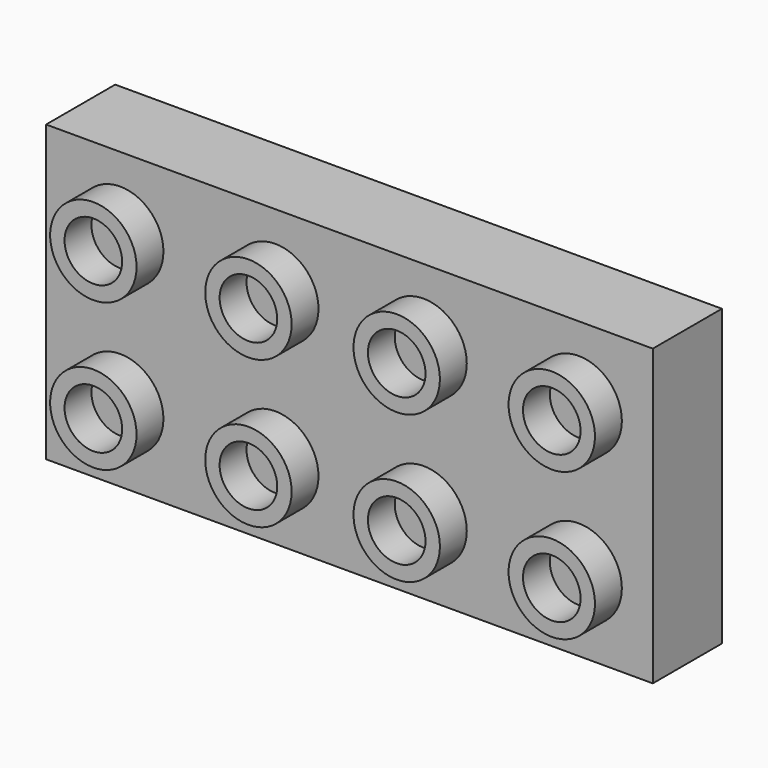
from build123d import *

# Parameters (mm, degrees)
F0_W     = 63.2
F0_H     = 30.7
F1_DEPTH = 9
F2_R     = 4.5
F2_R_2   = 3
F3_DEPTH = 3.5
F4_T     = 1


# Not quite as in the source:
# - a shell that OpenCascade refuses in one call is made with other operations: the cavity is built on its own and cut out


with BuildPart() as f1:
    # F0 (on Front) → F1 (new body)
    with BuildSketch(Plane.XZ):
        with Locations((2.7909118284, 0)):
            Rectangle(F0_W, F0_H)
    extrude(amount=F1_DEPTH)

    # F2 (on face) → F3 (join)
    with BuildSketch(Plane.XZ.offset(9)):
        with Locations((-21.0856401334, 7.675)):
            Circle(F2_R)
        with Locations((-21.0856401334, 7.675)):
            Circle(F2_R_2, mode=Mode.SUBTRACT)
        with Locations((-4.9325362097, 7.675)):
            Circle(F2_R)
        with Locations((-4.9325362097, 7.675)):
            Circle(F2_R_2, mode=Mode.SUBTRACT)
        with Locations((10.5143598666, 7.675)):
            Circle(F2_R)
        with Locations((10.5143598666, 7.675)):
            Circle(F2_R_2, mode=Mode.SUBTRACT)
        with Locations((-4.9325362097, -7.675)):
            Circle(F2_R)
        with Locations((-4.9325362097, -7.675)):
            Circle(F2_R_2, mode=Mode.SUBTRACT)
        with Locations((10.5143598666, -7.675)):
            Circle(F2_R)
        with Locations((10.5143598666, -7.675)):
            Circle(F2_R_2, mode=Mode.SUBTRACT)
        with Locations((-21.0856401334, -7.675)):
            Circle(F2_R)
        with Locations((-21.0856401334, -7.675)):
            Circle(F2_R_2, mode=Mode.SUBTRACT)
        with Locations((26.6674637903, -7.675)):
            Circle(F2_R)
        with Locations((26.6674637903, -7.675)):
            Circle(F2_R_2, mode=Mode.SUBTRACT)
        with Locations((26.6674637903, 7.675)):
            Circle(F2_R)
        with Locations((26.6674637903, 7.675)):
            Circle(F2_R_2, mode=Mode.SUBTRACT)
    extrude(amount=F3_DEPTH)

    # F4: shell of thickness 1, made by hand


with BuildPart() as f4_core1:
    # F4_t2: copy of F1
    add(f1.part)

    # the walls: a layer under each face that stays
    f4_faces = [f4_core1.faces().sort_by_distance(p)[0] for p in [
        (2.7909118284, -4.5, -15.35),
        (-28.8090881716, -4.5, 0),
        (34.3909118284, -4.5, 0),
        (2.7909118284, -9, 0),
        (2.7909118284, -4.5, 15.35),
        (-25.5856401334, -10.75, -7.675),
        (-9.4325362097, -10.75, -7.675),
        (6.0143598666, -10.75, -7.675),
        (22.1674637903, -10.75, -7.675),
        (-25.5856401334, -10.75, 7.675),
        (-9.4325362097, -10.75, 7.675),
        (6.0143598666, -10.75, 7.675),
        (22.1674637903, -10.75, 7.675),
        (-24.0856401334, -12.5, -10.675),
        (-7.9325362097, -12.5, -10.675),
        (7.5143598666, -12.5, -10.675),
        (23.6674637903, -12.5, -10.675),
        (-24.0856401334, -12.5, 4.675),
        (-7.9325362097, -12.5, 4.675),
        (7.5143598666, -12.5, 4.675),
        (23.6674637903, -12.5, 4.675),
        (-24.0856401334, -10.75, -7.675),
        (-7.9325362097, -10.75, -7.675),
        (7.5143598666, -10.75, -7.675),
        (23.6674637903, -10.75, -7.675),
        (-24.0856401334, -10.75, 7.675),
        (-7.9325362097, -10.75, 7.675),
        (7.5143598666, -10.75, 7.675),
        (23.6674637903, -10.75, 7.675),
        (-21.0856401334, -9, -7.675),
        (-4.9325362097, -9, -7.675),
        (10.5143598666, -9, -7.675),
        (26.6674637903, -9, -7.675),
        (-21.0856401334, -9, 7.675),
        (-4.9325362097, -9, 7.675),
        (10.5143598666, -9, 7.675),
        (26.6674637903, -9, 7.675),
    ]]
    thicken(f4_faces, amount=-F4_T, mode=Mode.SUBTRACT)

    # F4_s3 → F4_t4 (revolve, cut)
    with BuildSketch(Plane.XY.offset(-7.675)):
        Polygon((-16.5756401334, -9.01), (-16.5856401334, -8), (-17.5856401334, -8), (-17.5856401334, -9), align=None)
    revolve(axis=Axis((-21.0856401334, -9, -7.675), (0, -1, 0)), mode=Mode.SUBTRACT)

    # F4_s5 → F4_t6 (revolve, cut)
    with BuildSketch(Plane.XY.offset(-7.675)):
        Polygon((-0.4225362097, -9.01), (-0.4325362097, -8), (-1.4325362097, -8), (-1.4325362097, -9), align=None)
    revolve(axis=Axis((-4.9325362097, -9, -7.675), (0, -1, 0)), mode=Mode.SUBTRACT)

    # F4_s7 → F4_t8 (revolve, cut)
    with BuildSketch(Plane.XY.offset(-7.675)):
        Polygon((15.0243598666, -9.01), (15.0143598666, -8), (14.0143598666, -8), (14.0143598666, -9), align=None)
    revolve(axis=Axis((10.5143598666, -9, -7.675), (0, -1, 0)), mode=Mode.SUBTRACT)

    # F4_s9 → F4_t10 (revolve, cut)
    with BuildSketch(Plane.XY.offset(-7.675)):
        Polygon((31.1774637903, -9.01), (31.1674637903, -8), (30.1674637903, -8), (30.1674637903, -9), align=None)
    revolve(axis=Axis((26.6674637903, -9, -7.675), (0, -1, 0)), mode=Mode.SUBTRACT)

    # F4_s11 → F4_t12 (revolve, cut)
    with BuildSketch(Plane.XY.offset(7.675)):
        Polygon((-16.5756401334, -9.01), (-16.5856401334, -8), (-17.5856401334, -8), (-17.5856401334, -9), align=None)
    revolve(axis=Axis((-21.0856401334, -9, 7.675), (0, -1, 0)), mode=Mode.SUBTRACT)

    # F4_s13 → F4_t14 (revolve, cut)
    with BuildSketch(Plane.XY.offset(7.675)):
        Polygon((-0.4225362097, -9.01), (-0.4325362097, -8), (-1.4325362097, -8), (-1.4325362097, -9), align=None)
    revolve(axis=Axis((-4.9325362097, -9, 7.675), (0, -1, 0)), mode=Mode.SUBTRACT)

    # F4_s15 → F4_t16 (revolve, cut)
    with BuildSketch(Plane.XY.offset(7.675)):
        Polygon((15.0243598666, -9.01), (15.0143598666, -8), (14.0143598666, -8), (14.0143598666, -9), align=None)
    revolve(axis=Axis((10.5143598666, -9, 7.675), (0, -1, 0)), mode=Mode.SUBTRACT)

    # F4_s17 → F4_t18 (revolve, cut)
    with BuildSketch(Plane.XY.offset(7.675)):
        Polygon((31.1774637903, -9.01), (31.1674637903, -8), (30.1674637903, -8), (30.1674637903, -9), align=None)
    revolve(axis=Axis((26.6674637903, -9, 7.675), (0, -1, 0)), mode=Mode.SUBTRACT)

    # F4_s19 → F4_t20 (revolve, cut)
    with BuildSketch(Plane.XY.offset(-7.675)):
        Polygon((-18.0956401334, -9.01), (-17.0856401334, -9), (-17.0856401334, -8), (-18.0856401334, -8), align=None)
    revolve(axis=Axis((-21.0856401334, -9, -7.675), (0, -1, 0)), mode=Mode.SUBTRACT)

    # F4_s21 → F4_t22 (revolve, cut)
    with BuildSketch(Plane.XY.offset(-7.675)):
        Polygon((-1.9425362097, -9.01), (-0.9325362097, -9), (-0.9325362097, -8), (-1.9325362097, -8), align=None)
    revolve(axis=Axis((-4.9325362097, -9, -7.675), (0, -1, 0)), mode=Mode.SUBTRACT)

    # F4_s23 → F4_t24 (revolve, cut)
    with BuildSketch(Plane.XY.offset(-7.675)):
        Polygon((13.5043598666, -9.01), (14.5143598666, -9), (14.5143598666, -8), (13.5143598666, -8), align=None)
    revolve(axis=Axis((10.5143598666, -9, -7.675), (0, -1, 0)), mode=Mode.SUBTRACT)

    # F4_s25 → F4_t26 (revolve, cut)
    with BuildSketch(Plane.XY.offset(-7.675)):
        Polygon((29.6574637903, -9.01), (30.6674637903, -9), (30.6674637903, -8), (29.6674637903, -8), align=None)
    revolve(axis=Axis((26.6674637903, -9, -7.675), (0, -1, 0)), mode=Mode.SUBTRACT)

    # F4_s27 → F4_t28 (revolve, cut)
    with BuildSketch(Plane.XY.offset(7.675)):
        Polygon((-18.0956401334, -9.01), (-17.0856401334, -9), (-17.0856401334, -8), (-18.0856401334, -8), align=None)
    revolve(axis=Axis((-21.0856401334, -9, 7.675), (0, -1, 0)), mode=Mode.SUBTRACT)

    # F4_s29 → F4_t30 (revolve, cut)
    with BuildSketch(Plane.XY.offset(7.675)):
        Polygon((-1.9425362097, -9.01), (-0.9325362097, -9), (-0.9325362097, -8), (-1.9325362097, -8), align=None)
    revolve(axis=Axis((-4.9325362097, -9, 7.675), (0, -1, 0)), mode=Mode.SUBTRACT)

    # F4_s31 → F4_t32 (revolve, cut)
    with BuildSketch(Plane.XY.offset(7.675)):
        Polygon((13.5043598666, -9.01), (14.5143598666, -9), (14.5143598666, -8), (13.5143598666, -8), align=None)
    revolve(axis=Axis((10.5143598666, -9, 7.675), (0, -1, 0)), mode=Mode.SUBTRACT)

    # F4_s33 → F4_t34 (revolve, cut)
    with BuildSketch(Plane.XY.offset(7.675)):
        Polygon((29.6574637903, -9.01), (30.6674637903, -9), (30.6674637903, -8), (29.6674637903, -8), align=None)
    revolve(axis=Axis((26.6674637903, -9, 7.675), (0, -1, 0)), mode=Mode.SUBTRACT)


with BuildPart() as f1_1:
    add(f1.part)

    # what is left inside the walls is the cavity
    f4_cavity = [f4_core1.part.solids().sort_by_distance(p)[0] for p in [
        (2.790912, -0.01, -4.783333),
    ]]
    add(f4_cavity, mode=Mode.SUBTRACT)


solid = f1_1.part
